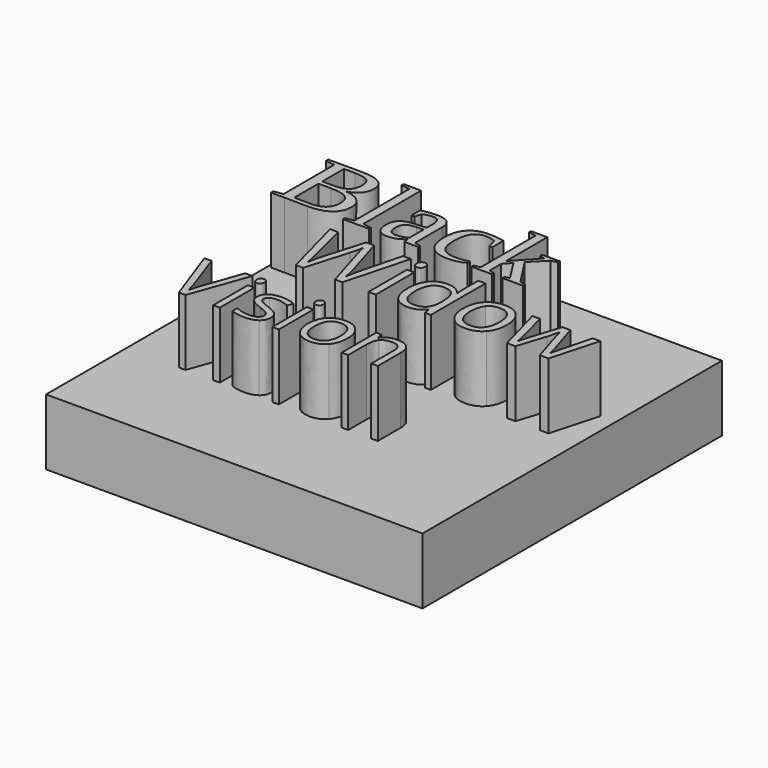
from build123d import *

# Parameters (mm, degrees)
F0_W         = 144.8050886393
F0_H         = 143.9752578735
F1_DEPTH     = 25.4
F2_TEXT_SIZE = 42.067695823
F3_DEPTH     = 25.4
F4_DEPTH     = 25.4
F2_W         = 2.8039144866
F2_H         = 18.5036745986
F5_DEPTH     = 25.4
F6_DEPTH     = 25.4
F7_DEPTH     = 25.4
F2_W_2       = 2.5235216114
F2_H_2       = 16.6532977245
F8_DEPTH     = 25.4
F9_DEPTH     = 25.4


# Not quite as in the source:
# - Text() gives the source's letters only with a copy of the font that has no kerning and outlines rounded to 1/6400 em; it was checked with that copy


with BuildPart() as f1:
    # F0 (on Top) → F1 (new body)
    with BuildSketch(Plane.XY):
        with Locations((1.0372623801, -2.489477396)):
            Rectangle(F0_W, F0_H)
    extrude(amount=F1_DEPTH)

    # F2 (on face) → F3 (join)
    with BuildSketch(Plane.XY.offset(25.4)):
        with Locations((-71.3652819395, 32.1558713913)):
            Text('Black', F2_TEXT_SIZE, font='Tinos', text_align=(TextAlign.LEFT, TextAlign.BOTTOM))
    extrude(amount=F3_DEPTH)

    # F2 (on face) → F4 (join)
    with BuildSketch(Plane.XY.offset(25.4)):
        with BuildLine():
            Line((-19.8046103162, 0), (-16.9682806332, 0))
            Line((-16.9682806332, 0), (-10.3663856377, 24.6841720412))
            Line((-10.3663856377, 24.6841720412), (-13.4080115644, 24.6841720412))
            Line((-13.4080115644, 24.6841720412), (-17.292432597, 9.4706398749))
            add(Edge.make_bspline(
                [(-18.5080024611, 3.6305019942), (-18.1838504973, 6.0292265262), (-17.292432597, 9.4706398749)],
                knots=[0, 0, 0, 1, 1, 1], degree=2))
            add(Edge.make_bspline(
                [(-19.8748432417, 9.5408728003), (-19.0644633322, 6.9206444265), (-18.5080024611, 3.6305019942)],
                knots=[0, 0, 0, 1, 1, 1], degree=2))
            Line((-19.8748432417, 9.5408728003), (-24.5156188563, 24.6841720412))
            Line((-24.5156188563, 24.6841720412), (-27.5572447831, 24.6841720412))
            Line((-27.5572447831, 24.6841720412), (-31.9765165558, 9.6759361186))
            add(Edge.make_bspline(
                [(-33.3271497382, 3.6305019942), (-32.8733369889, 6.7207507155), (-31.9765165558, 9.6759361186)],
                knots=[0, 0, 0, 1, 1, 1], degree=2))
            add(Edge.make_bspline(
                [(-34.510304406, 9.4382246785), (-33.6999244965, 6.2291202371), (-33.3271497382, 3.6305019942)],
                knots=[0, 0, 0, 1, 1, 1], degree=2))
            Line((-34.510304406, 9.4382246785), (-38.4109330367, 24.6841720412))
            Line((-38.4109330367, 24.6841720412), (-41.4525589634, 24.6841720412))
            Line((-41.4525589634, 24.6841720412), (-34.8830791643, 0))
            Line((-34.8830791643, 0), (-32.0467494813, 0))
            Line((-32.0467494813, 0), (-27.2168852211, 16.4291020305))
            add(Edge.make_bspline(
                [(-26.0337305533, 21.3075890853), (-26.4065053117, 19.076343068), (-27.2168852211, 16.4291020305)],
                knots=[0, 0, 0, 1, 1, 1], degree=2))
            add(Edge.make_bspline(
                [(-25.5799178041, 19.2978469099), (-26.0175229551, 20.9672295233), (-26.0337305533, 21.3075890853)],
                knots=[0, 0, 0, 1, 1, 1], degree=2))
            add(Edge.make_bspline(
                [(-24.7857454928, 16.5263476196), (-25.142312653, 17.6284642964), (-25.5799178041, 19.2978469099)],
                knots=[0, 0, 0, 1, 1, 1], degree=2))
            Line((-24.7857454928, 16.5263476196), (-19.8046103162, 0))
        make_face()
    extrude(amount=F4_DEPTH)

    # F2 (on face) → F5 (join)
    with BuildSketch(Plane.XY.offset(25.4)):
        with BuildLine():
            add(Edge.make_bspline(
                [(-7.1626837291, 23.5172249716), (-7.1626837291, 24.4788757975), (-6.6899621153, 24.927286014)],
                knots=[0, 0, 0, 1, 1, 1], degree=2))
            add(Edge.make_bspline(
                [(-6.6899621153, 22.1071639292), (-7.1626837291, 22.571781744), (-7.1626837291, 23.5172249716)],
                knots=[0, 0, 0, 1, 1, 1], degree=2))
            add(Edge.make_bspline(
                [(-5.5041061811, 21.6425461145), (-6.2172405014, 21.6425461145), (-6.6899621153, 22.1071639292)],
                knots=[0, 0, 0, 1, 1, 1], degree=2))
            add(Edge.make_bspline(
                [(-4.3398603779, 22.1071639292), (-4.8287895899, 21.6425461145), (-5.5041061811, 21.6425461145)],
                knots=[0, 0, 0, 1, 1, 1], degree=2))
            add(Edge.make_bspline(
                [(-3.8509311659, 23.5172249716), (-3.8509311659, 22.571781744), (-4.3398603779, 22.1071639292)],
                knots=[0, 0, 0, 1, 1, 1], degree=2))
            add(Edge.make_bspline(
                [(-4.3398603779, 24.9191822149), (-3.8509311659, 24.4626681993), (-3.8509311659, 23.5172249716)],
                knots=[0, 0, 0, 1, 1, 1], degree=2))
            add(Edge.make_bspline(
                [(-5.5041061811, 25.3756962306), (-4.8287895899, 25.3756962306), (-4.3398603779, 24.9191822149)],
                knots=[0, 0, 0, 1, 1, 1], degree=2))
            add(Edge.make_bspline(
                [(-6.6899621153, 24.927286014), (-6.2172405014, 25.3756962306), (-5.5041061811, 25.3756962306)],
                knots=[0, 0, 0, 1, 1, 1], degree=2))
        make_face()
        with Locations((-5.5230150457, 9.2518372993)):
            Rectangle(F2_W, F2_H)
        with BuildLine():
            Line((14.2637610762, 2.4797625229), (14.4150319926, 2.4797625229))
            Line((14.4150319926, 2.4797625229), (14.787806751, 0))
            Line((14.787806751, 0), (17.0676755628, 0))
            Line((17.0676755628, 0), (17.0676755628, 26.2725166637))
            Line((17.0676755628, 26.2725166637), (14.2637610762, 26.2725166637))
            Line((14.2637610762, 26.2725166637), (14.2637610762, 18.7413860387))
            Line((14.2637610762, 18.7413860387), (14.3339940017, 17.4393756509))
            Line((14.3339940017, 17.4393756509), (14.4528497217, 16.1049500667))
            Line((14.4528497217, 16.1049500667), (14.2313458798, 16.1049500667))
            add(Edge.make_bspline(
                [(8.456038392, 18.8440341606), (12.2216037044, 18.8440341606), (14.2313458798, 16.1049500667)],
                knots=[0, 0, 0, 1, 1, 1], degree=2))
            add(Edge.make_bspline(
                [(2.8157942223, 16.3102463104), (4.8417439959, 18.8440341606), (8.456038392, 18.8440341606)],
                knots=[0, 0, 0, 1, 1, 1], degree=2))
            add(Edge.make_bspline(
                [(0.7898444488, 9.2005132384), (0.7898444488, 13.7764584603), (2.8157942223, 16.3102463104)],
                knots=[0, 0, 0, 1, 1, 1], degree=2))
            add(Edge.make_bspline(
                [(2.8076904232, 2.1421042273), (0.7898444488, 4.6245680165), (0.7898444488, 9.2005132384)],
                knots=[0, 0, 0, 1, 1, 1], degree=2))
            add(Edge.make_bspline(
                [(8.456038392, -0.340359562), (4.8255363977, -0.340359562), (2.8076904232, 2.1421042273)],
                knots=[0, 0, 0, 1, 1, 1], degree=2))
            add(Edge.make_bspline(
                [(14.2637610762, 2.4797625229), (12.3242518263, -0.340359562), (8.456038392, -0.340359562)],
                knots=[0, 0, 0, 1, 1, 1], degree=2))
        make_face()
        with BuildLine():
            add(Edge.make_bspline(
                [(8.8126055521, 2.0097421754), (11.6813504315, 2.0097421754), (12.9725557539, 3.5710741342)],
                knots=[0, 0, 0, 1, 1, 1], degree=2))
            add(Edge.make_bspline(
                [(4.9957161787, 3.8168893734), (6.2950253002, 2.0097421754), (8.8126055521, 2.0097421754)],
                knots=[0, 0, 0, 1, 1, 1], degree=2))
            add(Edge.make_bspline(
                [(3.6964070573, 9.168098042), (3.6964070573, 5.6240365714), (4.9957161787, 3.8168893734)],
                knots=[0, 0, 0, 1, 1, 1], degree=2))
            add(Edge.make_bspline(
                [(5.0038199778, 14.5787345706), (3.6964070573, 12.663536718), (3.6964070573, 9.168098042)],
                knots=[0, 0, 0, 1, 1, 1], degree=2))
            add(Edge.make_bspline(
                [(8.7801903557, 16.4939324232), (6.3112328983, 16.4939324232), (5.0038199778, 14.5787345706)],
                knots=[0, 0, 0, 1, 1, 1], degree=2))
            add(Edge.make_bspline(
                [(12.9563481557, 14.8137447444), (11.6489352351, 16.4939324232), (8.7801903557, 16.4939324232)],
                knots=[0, 0, 0, 1, 1, 1], degree=2))
            add(Edge.make_bspline(
                [(14.2637610762, 9.2005132384), (14.2637610762, 13.1335570655), (12.9563481557, 14.8137447444)],
                knots=[0, 0, 0, 1, 1, 1], degree=2))
            Line((14.2637610762, 9.2005132384), (14.2637610762, 8.6116371709))
            add(Edge.make_bspline(
                [(12.9725557539, 3.5710741342), (14.2637610762, 5.1324060931), (14.2637610762, 8.6116371709)],
                knots=[0, 0, 0, 1, 1, 1], degree=2))
        make_face(mode=Mode.SUBTRACT)
    extrude(amount=F5_DEPTH)

    # F2 (on face) → F6 (join)
    with BuildSketch(Plane.XY.offset(25.4)):
        with BuildLine():
            add(Edge.make_bspline(
                [(38.9803483138, 9.2707461639), (38.9803483138, 4.7434237365), (36.7031807683, 2.2015320873)],
                knots=[0, 0, 0, 1, 1, 1], degree=2))
            add(Edge.make_bspline(
                [(36.6923757028, 16.2589222495), (38.9803483138, 13.6738103384), (38.9803483138, 9.2707461639)],
                knots=[0, 0, 0, 1, 1, 1], degree=2))
            add(Edge.make_bspline(
                [(30.5253845921, 18.8440341606), (34.4044030919, 18.8440341606), (36.6923757028, 16.2589222495)],
                knots=[0, 0, 0, 1, 1, 1], degree=2))
            add(Edge.make_bspline(
                [(24.2422390276, 16.3183501095), (26.5059002413, 18.8440341606), (30.5253845921, 18.8440341606)],
                knots=[0, 0, 0, 1, 1, 1], degree=2))
            add(Edge.make_bspline(
                [(21.978577814, 9.2707461639), (21.978577814, 13.7926660585), (24.2422390276, 16.3183501095)],
                knots=[0, 0, 0, 1, 1, 1], degree=2))
            add(Edge.make_bspline(
                [(23.0266691635, 4.1707552672), (21.978577814, 6.3479759572), (21.978577814, 9.2707461639)],
                knots=[0, 0, 0, 1, 1, 1], degree=2))
            add(Edge.make_bspline(
                [(25.9980621647, 0.8265875076), (24.074760513, 1.9935345772), (23.0266691635, 4.1707552672)],
                knots=[0, 0, 0, 1, 1, 1], degree=2))
            add(Edge.make_bspline(
                [(30.406528872, -0.340359562), (27.9213638165, -0.340359562), (25.9980621647, 0.8265875076)],
                knots=[0, 0, 0, 1, 1, 1], degree=2))
            add(Edge.make_bspline(
                [(36.7031807683, 2.2015320873), (34.4260132228, -0.340359562), (30.406528872, -0.340359562)],
                knots=[0, 0, 0, 1, 1, 1], degree=2))
        make_face()
        with BuildLine():
            add(Edge.make_bspline(
                [(24.8851404225, 9.2707461639), (24.8851404225, 5.7212821606), (26.303305264, 3.865512168)],
                knots=[0, 0, 0, 1, 1, 1], degree=2))
            add(Edge.make_bspline(
                [(26.2870976658, 14.6543700288), (24.8851404225, 12.8472228308), (24.8851404225, 9.2707461639)],
                knots=[0, 0, 0, 1, 1, 1], degree=2))
            add(Edge.make_bspline(
                [(30.4389440684, 16.4615172269), (27.6890549091, 16.4615172269), (26.2870976658, 14.6543700288)],
                knots=[0, 0, 0, 1, 1, 1], degree=2))
            add(Edge.make_bspline(
                [(34.6529195974, 14.6300586316), (33.2266509568, 16.4615172269), (30.4389440684, 16.4615172269)],
                knots=[0, 0, 0, 1, 1, 1], degree=2))
            add(Edge.make_bspline(
                [(36.079188238, 9.2707461639), (36.079188238, 12.7986000362), (34.6529195974, 14.6300586316)],
                knots=[0, 0, 0, 1, 1, 1], degree=2))
            add(Edge.make_bspline(
                [(34.6529195974, 3.8574083689), (36.079188238, 5.7050745624), (36.079188238, 9.2707461639)],
                knots=[0, 0, 0, 1, 1, 1], degree=2))
            add(Edge.make_bspline(
                [(30.4713592648, 2.0097421754), (33.2266509568, 2.0097421754), (34.6529195974, 3.8574083689)],
                knots=[0, 0, 0, 1, 1, 1], degree=2))
            add(Edge.make_bspline(
                [(26.303305264, 3.865512168), (27.7214701055, 2.0097421754), (30.4713592648, 2.0097421754)],
                knots=[0, 0, 0, 1, 1, 1], degree=2))
        make_face(mode=Mode.SUBTRACT)
    extrude(amount=F6_DEPTH)

    # F2 (on face) → F7 (join)
    with BuildSketch(Plane.XY.offset(25.4)):
        with BuildLine():
            Line((55.614746588, 10.8536882536), (59.0075371422, 0))
            Line((59.0075371422, 0), (62.3354973035, 0))
            Line((62.3354973035, 0), (67.4462932657, 18.5036745986))
            Line((67.4462932657, 18.5036745986), (64.5451331899, 18.5036745986))
            add(Edge.make_bspline(
                [(61.0253831166, 4.8811883211), (61.3198211504, 6.1480822462), (64.5451331899, 18.5036745986)],
                knots=[0, 0, 0, 1, 1, 1], degree=2))
            add(Edge.make_bspline(
                [(60.6607121574, 3.0038081976), (60.7309450829, 3.6142943961), (61.0253831166, 4.8811883211)],
                knots=[0, 0, 0, 1, 1, 1], degree=2))
            Line((60.6607121574, 3.0038081976), (60.5256488392, 3.0038081976))
            add(Edge.make_bspline(
                [(59.2452485823, 7.8822952524), (60.1906918099, 4.9811351766), (60.5256488392, 3.0038081976)],
                knots=[0, 0, 0, 1, 1, 1], degree=2))
            Line((59.2452485823, 7.8822952524), (55.9334960191, 18.5036745986))
            Line((55.9334960191, 18.5036745986), (52.8972726251, 18.5036745986))
            Line((52.8972726251, 18.5036745986), (49.5044820709, 7.8822952524))
            add(Edge.make_bspline(
                [(48.7832439515, 5.4619605896), (49.1965377053, 6.990877352), (49.5044820709, 7.8822952524)],
                knots=[0, 0, 0, 1, 1, 1], degree=2))
            add(Edge.make_bspline(
                [(48.1862640849, 2.9713930012), (48.3699501977, 3.9330438271), (48.7832439515, 5.4619605896)],
                knots=[0, 0, 0, 1, 1, 1], degree=2))
            Line((48.1862640849, 2.9713930012), (48.0512007667, 2.9713930012))
            add(Edge.make_bspline(
                [(46.9787980199, 7.8822952524), (47.9161374484, 4.2355856599), (48.0512007667, 2.9713930012)],
                knots=[0, 0, 0, 1, 1, 1], degree=2))
            add(Edge.make_bspline(
                [(44.2532202578, 18.5036745986), (46.0414585913, 11.5290048448), (46.9787980199, 7.8822952524)],
                knots=[0, 0, 0, 1, 1, 1], degree=2))
            Line((44.2532202578, 18.5036745986), (41.314242453, 18.5036745986))
            Line((41.314242453, 18.5036745986), (46.3602080223, 0))
            Line((46.3602080223, 0), (49.60172766, 0))
            Line((49.60172766, 0), (53.0971663361, 10.8212730572))
            add(Edge.make_bspline(
                [(54.2803210038, 15.381010681), (53.6050044126, 12.4258252779), (53.0971663361, 10.8212730572)],
                knots=[0, 0, 0, 1, 1, 1], degree=2))
            Line((54.2803210038, 15.381010681), (54.4153843221, 15.381010681))
            add(Edge.make_bspline(
                [(55.614746588, 10.8536882536), (55.2905946242, 11.8531568086), (54.4153843221, 15.381010681)],
                knots=[0, 0, 0, 1, 1, 1], degree=2))
        make_face()
    extrude(amount=F7_DEPTH)

    # F2 (on face) → F8 (join)
    with BuildSketch(Plane.XY.offset(25.4)):
        with BuildLine():
            Line((-40.604907143, -13.6743303059), (-43.3812671432, -13.6743303059))
            Line((-43.3812671432, -13.6743303059), (-48.4574840262, -27.9596992736))
            add(Edge.make_bspline(
                [(-49.8869933783, -32.8657364719), (-49.3375561103, -30.4054244577), (-48.4574840262, -27.9596992736)],
                knots=[0, 0, 0, 1, 1, 1], degree=2))
            add(Edge.make_bspline(
                [(-51.2824667935, -28.0472202543), (-50.4023947093, -30.5269813754), (-49.8869933783, -32.8657364719)],
                knots=[0, 0, 0, 1, 1, 1], degree=2))
            Line((-51.2824667935, -28.0472202543), (-56.3878573367, -13.6743303059))
            Line((-56.3878573367, -13.6743303059), (-59.1253191233, -13.6743303059))
            Line((-59.1253191233, -13.6743303059), (-51.1609098758, -35.8900725842))
            Line((-51.1609098758, -35.8900725842), (-48.6082146041, -35.8900725842))
            Line((-48.6082146041, -35.8900725842), (-40.604907143, -13.6743303059))
        make_face()
        with Locations((-36.6688941479, -27.5634237219)):
            Rectangle(F2_W_2, F2_H_2)
        with BuildLine():
            add(Edge.make_bspline(
                [(-38.1445951288, -14.7245820748), (-38.1445951288, -13.8590968208), (-37.7191459168, -13.455527854)],
                knots=[0, 0, 0, 1, 1, 1], degree=2))
            add(Edge.make_bspline(
                [(-37.7191459168, -15.9936362955), (-38.1445951288, -15.5754804986), (-38.1445951288, -14.7245820748)],
                knots=[0, 0, 0, 1, 1, 1], degree=2))
            add(Edge.make_bspline(
                [(-36.6518761794, -16.4117920924), (-37.2936967049, -16.4117920924), (-37.7191459168, -15.9936362955)],
                knots=[0, 0, 0, 1, 1, 1], degree=2))
            add(Edge.make_bspline(
                [(-35.6040555489, -15.9936362955), (-36.044091591, -16.4117920924), (-36.6518761794, -16.4117920924)],
                knots=[0, 0, 0, 1, 1, 1], degree=2))
            add(Edge.make_bspline(
                [(-35.1640195068, -14.7245820748), (-35.1640195068, -15.5754804986), (-35.6040555489, -15.9936362955)],
                knots=[0, 0, 0, 1, 1, 1], degree=2))
            add(Edge.make_bspline(
                [(-35.6040555489, -13.4628212691), (-35.1640195068, -13.8736836509), (-35.1640195068, -14.7245820748)],
                knots=[0, 0, 0, 1, 1, 1], degree=2))
            add(Edge.make_bspline(
                [(-36.6518761794, -13.0519588872), (-36.044091591, -13.0519588872), (-35.6040555489, -13.4628212691)],
                knots=[0, 0, 0, 1, 1, 1], degree=2))
            add(Edge.make_bspline(
                [(-37.7191459168, -13.455527854), (-37.2936967049, -13.0519588872), (-36.6518761794, -13.0519588872)],
                knots=[0, 0, 0, 1, 1, 1], degree=2))
        make_face()
        with BuildLine():
            add(Edge.make_bspline(
                [(-19.3178597159, -31.348706139), (-19.3178597159, -33.6728744054), (-21.0488302239, -34.9346352111)],
                knots=[0, 0, 0, 1, 1, 1], degree=2))
            add(Edge.make_bspline(
                [(-20.3583869313, -28.5966575223), (-19.3178597159, -29.6906697816), (-19.3178597159, -31.348706139)],
                knots=[0, 0, 0, 1, 1, 1], degree=2))
            add(Edge.make_bspline(
                [(-24.3600406619, -26.4232198339), (-21.3989141468, -27.5026452631), (-20.3583869313, -28.5966575223)],
                knots=[0, 0, 0, 1, 1, 1], degree=2))
            add(Edge.make_bspline(
                [(-27.2774066867, -25.1906326885), (-26.5188915202, -25.6160819004), (-24.3600406619, -26.4232198339)],
                knots=[0, 0, 0, 1, 1, 1], degree=2))
            add(Edge.make_bspline(
                [(-28.378712361, -24.2959737742), (-28.0359218531, -24.7651834765), (-27.2774066867, -25.1906326885)],
                knots=[0, 0, 0, 1, 1, 1], degree=2))
            add(Edge.make_bspline(
                [(-28.7215028689, -23.1557698862), (-28.7215028689, -23.8267640719), (-28.378712361, -24.2959737742)],
                knots=[0, 0, 0, 1, 1, 1], degree=2))
            add(Edge.make_bspline(
                [(-27.8098259862, -21.6071347548), (-28.7215028689, -22.1687277145), (-28.7215028689, -23.1557698862)],
                knots=[0, 0, 0, 1, 1, 1], degree=2))
            add(Edge.make_bspline(
                [(-25.1039689982, -21.045541795), (-26.8981491034, -21.045541795), (-27.8098259862, -21.6071347548)],
                knots=[0, 0, 0, 1, 1, 1], degree=2))
            add(Edge.make_bspline(
                [(-20.5626025531, -22.0763444571), (-23.0666750576, -21.045541795), (-25.1039689982, -21.045541795)],
                knots=[0, 0, 0, 1, 1, 1], degree=2))
            Line((-20.5626025531, -22.0763444571), (-19.6630813621, -20.0244636863))
            add(Edge.make_bspline(
                [(-24.92406476, -18.9304514271), (-22.2352257406, -18.9304514271), (-19.6630813621, -20.0244636863)],
                knots=[0, 0, 0, 1, 1, 1], degree=2))
            add(Edge.make_bspline(
                [(-29.4654312052, -20.1095535287), (-27.8073948478, -18.9304514271), (-24.92406476, -18.9304514271)],
                knots=[0, 0, 0, 1, 1, 1], degree=2))
            add(Edge.make_bspline(
                [(-31.1234675626, -23.325949571), (-31.1234675626, -21.2886556304), (-29.4654312052, -20.1095535287)],
                knots=[0, 0, 0, 1, 1, 1], degree=2))
            add(Edge.make_bspline(
                [(-30.6445333069, -25.2830159459), (-31.1234675626, -24.4637223206), (-31.1234675626, -23.325949571)],
                knots=[0, 0, 0, 1, 1, 1], degree=2))
            add(Edge.make_bspline(
                [(-29.1858502945, -26.7489923733), (-30.1655990511, -26.1023095712), (-30.6445333069, -25.2830159459)],
                knots=[0, 0, 0, 1, 1, 1], degree=2))
            add(Edge.make_bspline(
                [(-25.8819332715, -28.2611604295), (-28.2061015379, -27.3956751755), (-29.1858502945, -26.7489923733)],
                knots=[0, 0, 0, 1, 1, 1], degree=2))
            add(Edge.make_bspline(
                [(-22.5901719403, -29.8948854033), (-23.4313458107, -29.2044421108), (-25.8819332715, -28.2611604295)],
                knots=[0, 0, 0, 1, 1, 1], degree=2))
            add(Edge.make_bspline(
                [(-21.7489980698, -31.5577840374), (-21.7489980698, -30.5853286959), (-22.5901719403, -29.8948854033)],
                knots=[0, 0, 0, 1, 1, 1], degree=2))
            add(Edge.make_bspline(
                [(-22.8114055305, -33.4808144754), (-21.7489980698, -32.8511496417), (-21.7489980698, -31.5577840374)],
                knots=[0, 0, 0, 1, 1, 1], degree=2))
            add(Edge.make_bspline(
                [(-25.8478973345, -34.1104793091), (-23.8738129911, -34.1104793091), (-22.8114055305, -33.4808144754)],
                knots=[0, 0, 0, 1, 1, 1], degree=2))
            add(Edge.make_bspline(
                [(-28.5002692787, -33.7628265245), (-27.1266761087, -34.1104793091), (-25.8478973345, -34.1104793091)],
                knots=[0, 0, 0, 1, 1, 1], degree=2))
            add(Edge.make_bspline(
                [(-31.0748447955, -32.8073891514), (-29.8738624487, -33.4151737398), (-28.5002692787, -33.7628265245)],
                knots=[0, 0, 0, 1, 1, 1], degree=2))
            Line((-31.0748447955, -32.8073891514), (-31.0748447955, -35.1461442478))
            add(Edge.make_bspline(
                [(-25.9111069317, -36.1963960167), (-29.2223173698, -36.1963960167), (-31.0748447955, -35.1461442478)],
                knots=[0, 0, 0, 1, 1, 1], degree=2))
            add(Edge.make_bspline(
                [(-21.0488302239, -34.9346352111), (-22.7798007319, -36.1963960167), (-25.9111069317, -36.1963960167)],
                knots=[0, 0, 0, 1, 1, 1], degree=2))
        make_face()
        with BuildLine():
            add(Edge.make_bspline(
                [(-15.4280383496, -14.7245820748), (-15.4280383496, -13.8590968208), (-15.0025891376, -13.455527854)],
                knots=[0, 0, 0, 1, 1, 1], degree=2))
            add(Edge.make_bspline(
                [(-15.0025891376, -15.9936362955), (-15.4280383496, -15.5754804986), (-15.4280383496, -14.7245820748)],
                knots=[0, 0, 0, 1, 1, 1], degree=2))
            add(Edge.make_bspline(
                [(-13.9353194002, -16.4117920924), (-14.5771399257, -16.4117920924), (-15.0025891376, -15.9936362955)],
                knots=[0, 0, 0, 1, 1, 1], degree=2))
            add(Edge.make_bspline(
                [(-12.8874987697, -15.9936362955), (-13.3275348118, -16.4117920924), (-13.9353194002, -16.4117920924)],
                knots=[0, 0, 0, 1, 1, 1], degree=2))
            add(Edge.make_bspline(
                [(-12.4474627276, -14.7245820748), (-12.4474627276, -15.5754804986), (-12.8874987697, -15.9936362955)],
                knots=[0, 0, 0, 1, 1, 1], degree=2))
            add(Edge.make_bspline(
                [(-12.8874987697, -13.4628212691), (-12.4474627276, -13.8736836509), (-12.4474627276, -14.7245820748)],
                knots=[0, 0, 0, 1, 1, 1], degree=2))
            add(Edge.make_bspline(
                [(-13.9353194002, -13.0519588872), (-13.3275348118, -13.0519588872), (-12.8874987697, -13.4628212691)],
                knots=[0, 0, 0, 1, 1, 1], degree=2))
            add(Edge.make_bspline(
                [(-15.0025891376, -13.455527854), (-14.5771399257, -13.0519588872), (-13.9353194002, -13.0519588872)],
                knots=[0, 0, 0, 1, 1, 1], degree=2))
        make_face()
        with Locations((-13.9523373687, -27.5634237219)):
            Rectangle(F2_W_2, F2_H_2)
        with BuildLine():
            add(Edge.make_bspline(
                [(7.0308177641, -27.5464057534), (7.0308177641, -31.6209936346), (4.9813681318, -33.9086948257)],
                knots=[0, 0, 0, 1, 1, 1], degree=2))
            add(Edge.make_bspline(
                [(4.9716435784, -21.2570508318), (7.0308177641, -23.5836502365), (7.0308177641, -27.5464057534)],
                knots=[0, 0, 0, 1, 1, 1], degree=2))
            add(Edge.make_bspline(
                [(-0.5786452837, -18.9304514271), (2.9124693926, -18.9304514271), (4.9716435784, -21.2570508318)],
                knots=[0, 0, 0, 1, 1, 1], degree=2))
            add(Edge.make_bspline(
                [(-6.233473095, -21.203565788), (-4.1961791544, -18.9304514271), (-0.5786452837, -18.9304514271)],
                knots=[0, 0, 0, 1, 1, 1], degree=2))
            add(Edge.make_bspline(
                [(-8.2707670356, -27.5464057534), (-8.2707670356, -23.4766801489), (-6.233473095, -21.203565788)],
                knots=[0, 0, 0, 1, 1, 1], degree=2))
            add(Edge.make_bspline(
                [(-7.3274853542, -32.1363949657), (-8.2707670356, -30.1768974524), (-8.2707670356, -27.5464057534)],
                knots=[0, 0, 0, 1, 1, 1], degree=2))
            add(Edge.make_bspline(
                [(-4.6532331649, -35.1461442478), (-6.3842036729, -34.0958924789), (-7.3274853542, -32.1363949657)],
                knots=[0, 0, 0, 1, 1, 1], degree=2))
            add(Edge.make_bspline(
                [(-0.6856153713, -36.1963960167), (-2.9222626569, -36.1963960167), (-4.6532331649, -35.1461442478)],
                knots=[0, 0, 0, 1, 1, 1], degree=2))
            add(Edge.make_bspline(
                [(4.9813681318, -33.9086948257), (2.9319184994, -36.1963960167), (-0.6856153713, -36.1963960167)],
                knots=[0, 0, 0, 1, 1, 1], degree=2))
        make_face()
        with BuildLine():
            add(Edge.make_bspline(
                [(-5.6548621667, -27.5464057534), (-5.6548621667, -30.7409215505), (-4.3785145309, -32.4111135997)],
                knots=[0, 0, 0, 1, 1, 1], degree=2))
            add(Edge.make_bspline(
                [(-4.393101361, -22.701147014), (-5.6548621667, -24.3275785728), (-5.6548621667, -27.5464057534)],
                knots=[0, 0, 0, 1, 1, 1], degree=2))
            add(Edge.make_bspline(
                [(-0.656441711, -21.0747154552), (-3.1313405553, -21.0747154552), (-4.393101361, -22.701147014)],
                knots=[0, 0, 0, 1, 1, 1], degree=2))
            add(Edge.make_bspline(
                [(3.1361341211, -22.7230272592), (1.8524930702, -21.0747154552), (-0.656441711, -21.0747154552)],
                knots=[0, 0, 0, 1, 1, 1], degree=2))
            add(Edge.make_bspline(
                [(4.419775172, -27.5464057534), (4.419775172, -24.3713390632), (3.1361341211, -22.7230272592)],
                knots=[0, 0, 0, 1, 1, 1], degree=2))
            add(Edge.make_bspline(
                [(3.1361341211, -32.4184070147), (4.419775172, -30.7555083806), (4.419775172, -27.5464057534)],
                knots=[0, 0, 0, 1, 1, 1], degree=2))
            add(Edge.make_bspline(
                [(-0.6272680508, -34.0813056488), (1.8524930702, -34.0813056488), (3.1361341211, -32.4184070147)],
                knots=[0, 0, 0, 1, 1, 1], degree=2))
            add(Edge.make_bspline(
                [(-4.3785145309, -32.4111135997), (-3.1021668951, -34.0813056488), (-0.6272680508, -34.0813056488)],
                knots=[0, 0, 0, 1, 1, 1], degree=2))
        make_face(mode=Mode.SUBTRACT)
    extrude(amount=F8_DEPTH)

    # F2 (on face) → F9 (join)
    with BuildSketch(Plane.XY.offset(25.4)):
        with BuildLine():
            Line((22.8526661716, -25.1152673995), (22.8526661716, -35.8900725842))
            Line((22.8526661716, -35.8900725842), (25.376187783, -35.8900725842))
            Line((25.376187783, -35.8900725842), (25.376187783, -25.0277464187))
            add(Edge.make_bspline(
                [(23.8567263118, -20.3818410244), (25.376187783, -21.8332306217), (25.376187783, -25.0277464187)],
                knots=[0, 0, 0, 1, 1, 1], degree=2))
            add(Edge.make_bspline(
                [(19.3275155584, -18.9304514271), (22.3372648405, -18.9304514271), (23.8567263118, -20.3818410244)],
                knots=[0, 0, 0, 1, 1, 1], degree=2))
            add(Edge.make_bspline(
                [(16.213227327, -19.6087390278), (17.6111318805, -18.9304514271), (19.3275155584, -18.9304514271)],
                knots=[0, 0, 0, 1, 1, 1], degree=2))
            add(Edge.make_bspline(
                [(14.0373585002, -21.5171826357), (14.8153227735, -20.2870266286), (16.213227327, -19.6087390278)],
                knots=[0, 0, 0, 1, 1, 1], degree=2))
            Line((14.0373585002, -21.5171826357), (13.9158015825, -21.5171826357))
            Line((13.9158015825, -21.5171826357), (13.507370339, -19.2367748597))
            Line((13.507370339, -19.2367748597), (11.4554895683, -19.2367748597))
            Line((11.4554895683, -19.2367748597), (11.4554895683, -35.8900725842))
            Line((11.4554895683, -35.8900725842), (13.9790111797, -35.8900725842))
            Line((13.9790111797, -35.8900725842), (13.9790111797, -27.1525613401))
            add(Edge.make_bspline(
                [(15.1945803567, -22.4872068389), (13.9790111797, -23.8996982225), (13.9790111797, -27.1525613401)],
                knots=[0, 0, 0, 1, 1, 1], degree=2))
            add(Edge.make_bspline(
                [(19.0211921258, -21.0747154552), (16.4101495336, -21.0747154552), (15.1945803567, -22.4872068389)],
                knots=[0, 0, 0, 1, 1, 1], degree=2))
            add(Edge.make_bspline(
                [(21.9264024587, -22.0787755954), (21.0001387459, -21.0747154552), (19.0211921258, -21.0747154552)],
                knots=[0, 0, 0, 1, 1, 1], degree=2))
            add(Edge.make_bspline(
                [(22.8526661716, -25.1152673995), (22.8526661716, -23.0828357356), (21.9264024587, -22.0787755954)],
                knots=[0, 0, 0, 1, 1, 1], degree=2))
        make_face()
    extrude(amount=F9_DEPTH)


solid = f1.part
